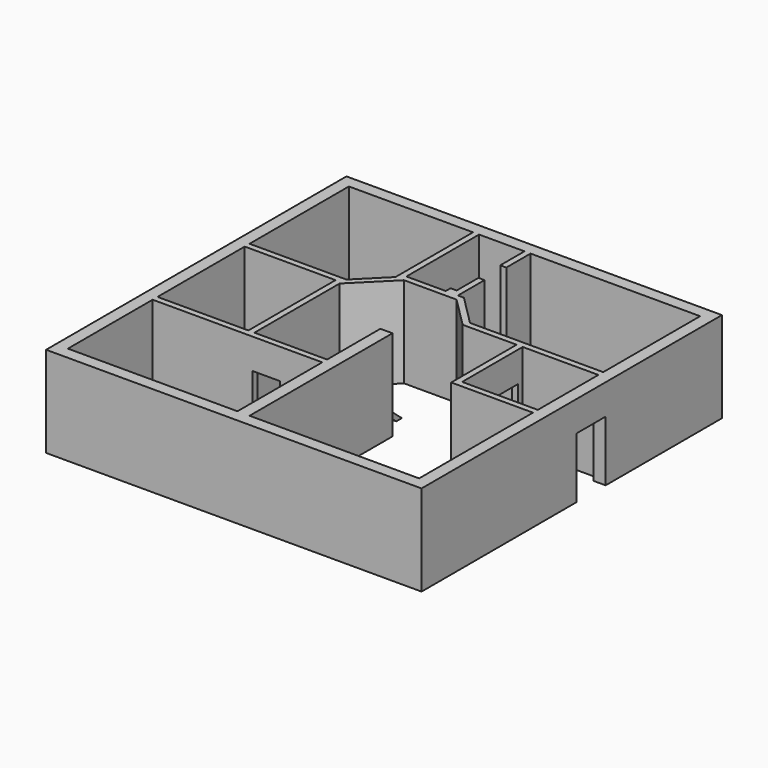
from build123d import *

# Parameters (mm, degrees)
F0_W      = 12400
F0_H      = 12400
F1_DEPTH  = 3000
F2_W      = 1200
F2_H      = 2000
F3_DEPTH  = 6000
F4_W      = 1300
F4_H      = 2000
F5_DEPTH  = 2800
F6_W      = 900
F6_H      = 2000
F7_DEPTH  = 200
F10_DEPTH = 900


# Not quite as in the source:
# - a feature names something its author has since deleted; it is built from what else it names


with BuildPart() as f1:
    # F0 (on Top) → F1 (new body)
    with BuildSketch(Plane.XY):
        with Locations((6200, 6200)):
            Rectangle(F0_W, F0_H)
        Polygon((6000, 400), (400, 400), (400, 3900), (400, 4100), (400, 7700), (400, 7900), (400, 12000), (4500, 12000), (4700, 12000), (6000, 12000), (6200, 12000), (6200, 11000), (6400, 11000), (6400, 12000), (12000, 12000), (12000, 8000), (12000, 7800), (12000, 5300), (12000, 5100), (12000, 400), (6400, 400), (6400, 6300), (6000, 6300), (6000, 4100), (6000, 3900), align=None, mode=Mode.SUBTRACT)
        Polygon((400, 7900), (400, 7700), (3400, 7700), (3400, 4100), (3600, 4100), (3600, 7617.1572875254), (4782.8427124746, 8800), (6517.1572875254, 8800), (7517.1572875254, 7800), (9300, 7800), (9300, 5100), (12000, 5100), (12000, 5300), (9500, 5300), (9500, 7800), (12000, 7800), (12000, 8000), (7600, 8000), (6600, 9000), (6400, 9000), (6400, 10100), (6200, 10100), (6200, 9200), (6000, 9200), (6000, 9000), (4700, 9000), (4700, 12000), (4500, 12000), (4500, 8800), (3600, 7900), align=None)
        Polygon((400, 4100), (400, 3900), (6000, 3900), (6000, 4100), (3600, 4100), (3400, 4100), align=None)
    extrude(amount=F1_DEPTH)

    # F2 (on face) → F3 (cut, through all)
    with BuildSketch(Plane.YZ.offset(12400)):
        with Locations((7000, 1000)):
            Rectangle(F2_W, F2_H)
    extrude(amount=-F3_DEPTH, mode=Mode.SUBTRACT)

    # F4 (on face) → F5 (cut, through all)
    with BuildSketch(Plane.YZ.offset(6400)):
        with Locations((6950, 1000)):
            Rectangle(F4_W, F4_H)
    extrude(amount=-F5_DEPTH, mode=Mode.SUBTRACT)

    # F6 (on face) → F7 (cut, through all)
    with BuildSketch(Plane(origin=(0, 4100, 0), x_dir=(-1, 0, 0), z_dir=(0, 1, 0))):
        with Locations((-4150, 1000)):
            Rectangle(F6_W, F6_H)
    extrude(amount=-F7_DEPTH, mode=Mode.SUBTRACT)


with BuildPart() as f10:
    # F9 (on plane+point) → F10 (new body)
    with BuildSketch(Plane(origin=(5950, 0, 0), x_dir=(0, -1, 0), z_dir=(-1, 0, 0))):
        Polygon((-4866.4928148116, 2000), (-7250, 0), (-7016.6414259709, 0), (-4866.4928148116, 1804.1889066002), align=None)
    extrude(amount=F10_DEPTH)


solid = Compound([f1.part, f10.part])
